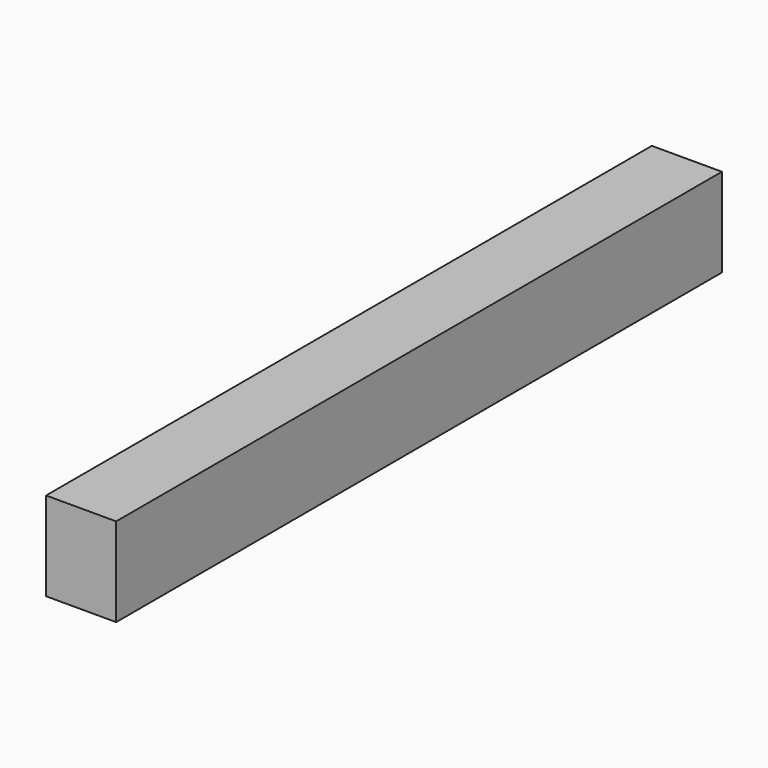
from build123d import *

# Parameters (mm, degrees)
F0_W     = 40.1181057096
F0_H     = 433.4320127964
F1_DEPTH = 25.4
F2_W     = 40.1181057096
F2_H     = 433.4320127964
F3_DEPTH = 25.4


# Not quite as in the source:
# - the program builds the solid bodies; features that only make, move or delete a surface that nothing else refers to are left out


with BuildPart() as f1:
    # F0 (on Top) → F1 (new body)
    with BuildSketch(Plane.XY):
        with Locations((-20.0590528548, -142.2124505043)):
            Rectangle(F0_W, F0_H)
    extrude(amount=F1_DEPTH)

    # F2 (on face) → F3 (join)
    with BuildSketch(Plane.XY.offset(25.4)):
        with Locations((-20.0590528548, -142.2124505043)):
            Rectangle(F2_W, F2_H)
    extrude(amount=F3_DEPTH)


solid = f1.part
